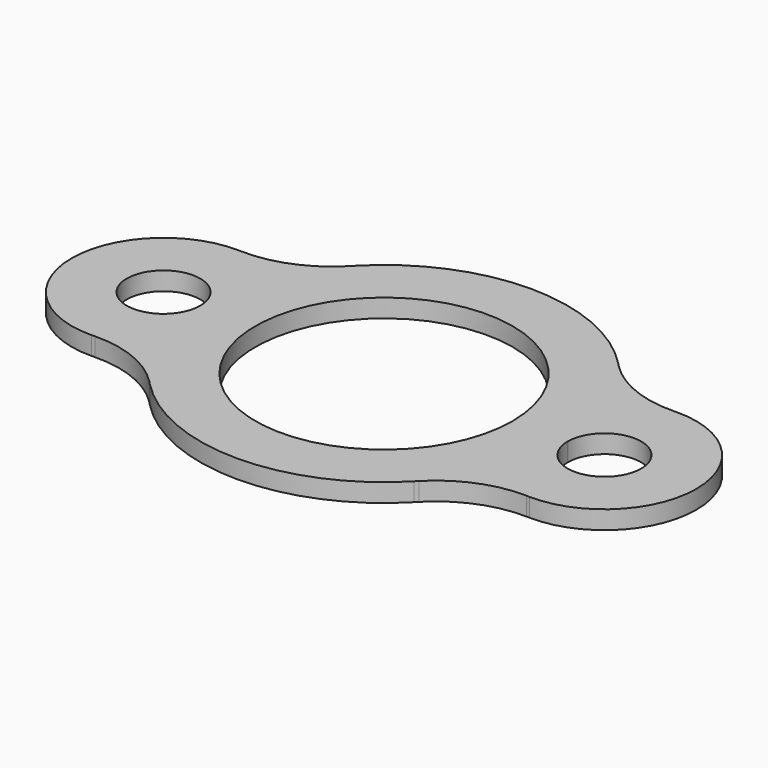
from build123d import *

# Parameters (mm, degrees)
F0_R     = 12.7
F0_R_2   = 44.45
F1_DEPTH = 6.35


# Not quite as in the source:
# - a length typed as a fraction of an inch, garbled in the dataset ("3 / 203.2 mm" for 3/8 in), is restored


with BuildPart() as f1:
    # F0 (on Top) → F1 (new body)
    with BuildSketch(Plane.XY):
        with BuildLine():
            ThreePointArc((-74.5464027897, -31.7069095982), (-59.4196204119, -34.5232781397), (-46.6403597532, -43.0931074194))
            ThreePointArc((-46.6403597532, -43.0931074194), (-46.1303112619, -43.6221670242), (-45.6305618227, -44.160965713))
            ThreePointArc((-45.6305618227, -44.160965713), (0, -63.500701295), (45.6305618227, -44.160965713))
            ThreePointArc((45.6305618227, -44.160965713), (46.1303112619, -43.6221670242), (46.6403597532, -43.0931074194))
            ThreePointArc((46.6403597532, -43.0931074194), (59.4196204119, -34.5232781397), (74.5464027897, -31.7069095982))
            ThreePointArc((74.5464027897, -31.7069095982), (75.115235957, -31.7221094671), (75.6837786723, -31.745803117))
            ThreePointArc((75.6837786723, -31.745803117), (107.95, 0), (75.6837786723, 31.745803117))
            ThreePointArc((75.6837786723, 31.745803117), (75.115235957, 31.7221094671), (74.5464027897, 31.7069095982))
            ThreePointArc((74.5464027897, 31.7069095982), (59.4196204119, 34.5232781397), (46.6403597532, 43.0931074194))
            ThreePointArc((46.6403597532, 43.0931074194), (46.1303112619, 43.6221670242), (45.6305618227, 44.160965713))
            ThreePointArc((45.6305618227, 44.160965713), (0, 63.500701295), (-45.6305618227, 44.160965713))
            ThreePointArc((-45.6305618227, 44.160965713), (-46.1303112619, 43.6221670242), (-46.6403597532, 43.0931074194))
            ThreePointArc((-46.6403597532, 43.0931074194), (-59.4196204119, 34.5232781397), (-74.5464027897, 31.7069095982))
            ThreePointArc((-74.5464027897, 31.7069095982), (-75.115235957, 31.7221094671), (-75.6837786723, 31.745803117))
            ThreePointArc((-75.6837786723, 31.745803117), (-107.95, 0), (-75.6837786723, -31.745803117))
            ThreePointArc((-75.6837786723, -31.745803117), (-75.115235957, -31.7221094671), (-74.5464027897, -31.7069095982))
        make_face()
        with Locations((-76.2, 0)):
            Circle(F0_R, mode=Mode.SUBTRACT)
        Circle(F0_R_2, mode=Mode.SUBTRACT)
        with BuildLine():
            ThreePointArc((63.5005844158, 0.1218352114), (76.2609183065, 12.6998538952), (88.9, 0))
            ThreePointArc((88.9, 0), (76.2609183065, -12.6998538952), (63.5005844158, -0.1218352114))
            ThreePointArc((63.5005844158, -0.1218352114), (63.5, 0), (63.5005844158, 0.1218352114))
        make_face(mode=Mode.SUBTRACT)
    extrude(amount=F1_DEPTH)


solid = f1.part
